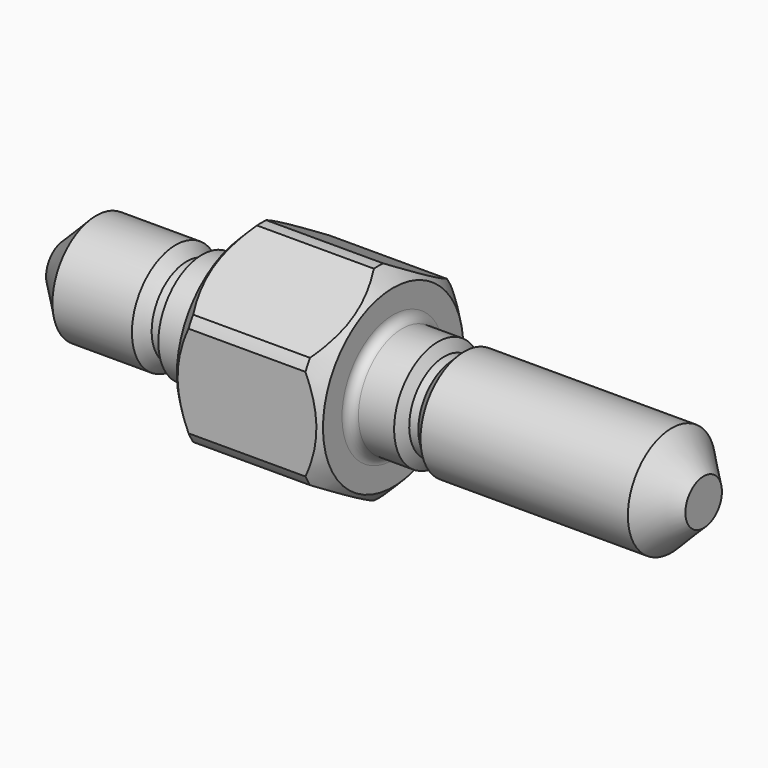
from build123d import *

# Parameters (mm, degrees)
F2_R     = 12.5
F3_DEPTH = 12.5
F4_R     = 0.5


# Not quite as in the source:
# - the program builds the solid bodies; features that only make, move or delete a surface that nothing else refers to are left out


with BuildPart() as f1:
    # F0 (on Front) → F1 (revolve)
    with BuildSketch(Plane.XZ):
        Polygon((-14, 0), (21, 0), (21, 1.25), (19.85, 2.4), (7.3, 2.4), (6.8, 2.4), (6.4535898385, 3), (4, 3), (4, 4.8), (3.2, 5.6), (-3.2, 5.6), (-4, 4.8), (-4, 3), (-6.4535898385, 3), (-6.8, 2.4), (-7.3, 2.4), (-12.85, 2.4), (-14, 1.25), align=None)
        Polygon((7.3, 2.4), (19.85, 2.4), (19.25, 3), (7.9, 3), align=None)
        Polygon((-12.25, 3), (-12.85, 2.4), (-7.3, 2.4), (-7.9, 3), align=None)
    revolve(axis=Axis((0, 0, 0), (1, 0, 0)))

    # F2 (on Right) → F3 (cut, symmetric)
    with BuildSketch(Plane.YZ):
        Circle(F2_R)
        Polygon((5, -2.8867513459), (0, -5.7735026919), (-5, -2.8867513459), (-5, 2.8867513459), (0, 5.7735026919), (5, 2.8867513459), align=None, mode=Mode.SUBTRACT)
    extrude(amount=F3_DEPTH, both=True, mode=Mode.SUBTRACT)

    # F4
    f4_edges = [f1.edges().sort_by_distance(p)[0] for p in [
        (-4, 0, -3),
        (4, 0, -3),
    ]]
    fillet(f4_edges, radius=F4_R)


solid = f1.part
